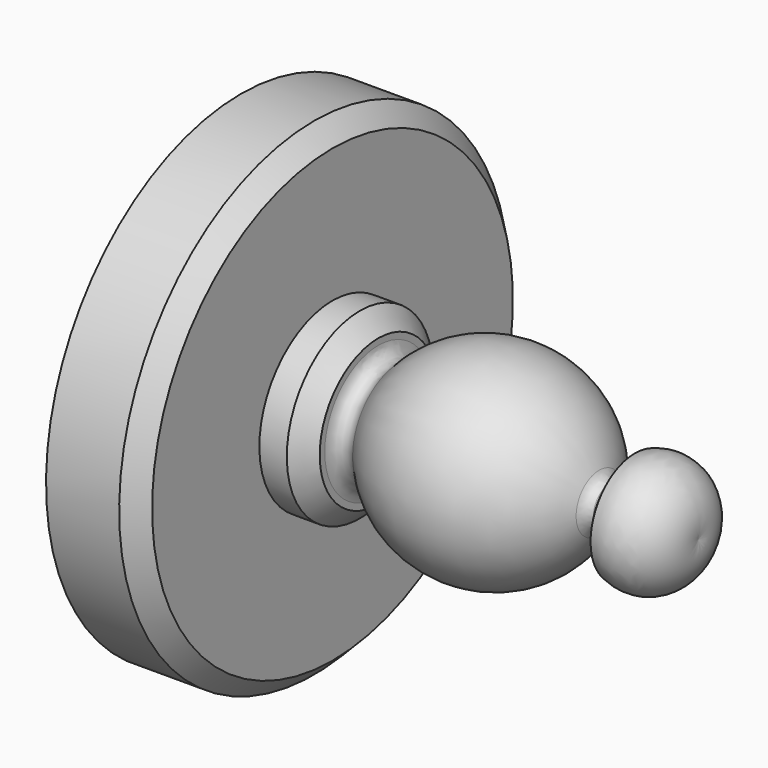
from build123d import *

# Parameters (mm, degrees)
F2_R = 0.508


# Not quite as in the source:
# - a fillet or chamfer that OpenCascade refuses, or shapes differently, is made with other operations: its cross-section is extruded or revolved along the edge and cut away or added


with BuildPart() as f1:
    # F0 (on Front) → F1 (revolve)
    with BuildSketch(Plane.XZ):
        with BuildLine():
            Line((-19.05, 0), (0, 0))
            ThreePointArc((0, 0), (-0.8365584984, 2.1276164223), (-3.1208319045, 2.034467252))
            Line((-3.1208319045, 2.034467252), (-3.1208319045, 0.891467252))
            Line((-3.1208319045, 0.891467252), (-4.0098319045, 0.891467252))
            ThreePointArc((-4.0098319045, 0.891467252), (-8.6732915332, 4.1995590152), (-13.335, 0.889))
            Line((-13.335, 0.889), (-13.335, 3.81))
            Line((-13.335, 3.81), (-15.24, 3.81))
            Line((-15.24, 3.81), (-15.24, 10.16))
            Line((-15.24, 10.16), (-19.05, 10.16))
            Line((-19.05, 10.16), (-19.05, 0))
        make_face()
    revolve(axis=Axis((-9.525, 0, 0), (-1, 0, 0)))

    # F2
    f2_edges = [f1.edges().sort_by_distance(p)[0] for p in [
        (-4.009832, 0, -0.891467),
        (-13.335, 0, -0.889),
        (-8.673292, 0, 4.199559),
    ]]
    fillet(f2_edges, radius=F2_R)

    # F3: chamfer of 0.762 on 3 edges, made by hand

    # F3_s1 → F3_t2 (revolve, cut)
    with BuildSketch(Plane.XZ):
        Polygon((-15.24, 9.398), (-16.002, 10.16), (-15.24, 10.16), align=None)
    revolve(axis=Axis((-15.24, 0, 0), (-1, 0, 0)), mode=Mode.SUBTRACT)

    # F3_s3 → F3_t4 (revolve, cut)
    with BuildSketch(Plane.XZ):
        Polygon((-13.335, 3.048), (-14.097, 3.81), (-13.335, 3.81), align=None)
    revolve(axis=Axis((-13.335, 0, 0), (-1, 0, 0)), mode=Mode.SUBTRACT)

    # F3_s5 → F3_t6 (revolve, cut)
    with BuildSketch(Plane.XZ):
        with BuildLine():
            Line((-3.1208319045, 1.600505207), (-2.6395418811, 2.3089160405))
            ThreePointArc((-2.6395418811, 2.3089160405), (-2.8778866419, 2.1954632748), (-3.1208319045, 2.034467252))
            Line((-3.1208319045, 2.034467252), (-3.1208319045, 1.600505207))
        make_face()
    revolve(axis=Axis((-3.1208319045, 0, 0), (-1, 0, 0)), mode=Mode.SUBTRACT)


solid = f1.part
